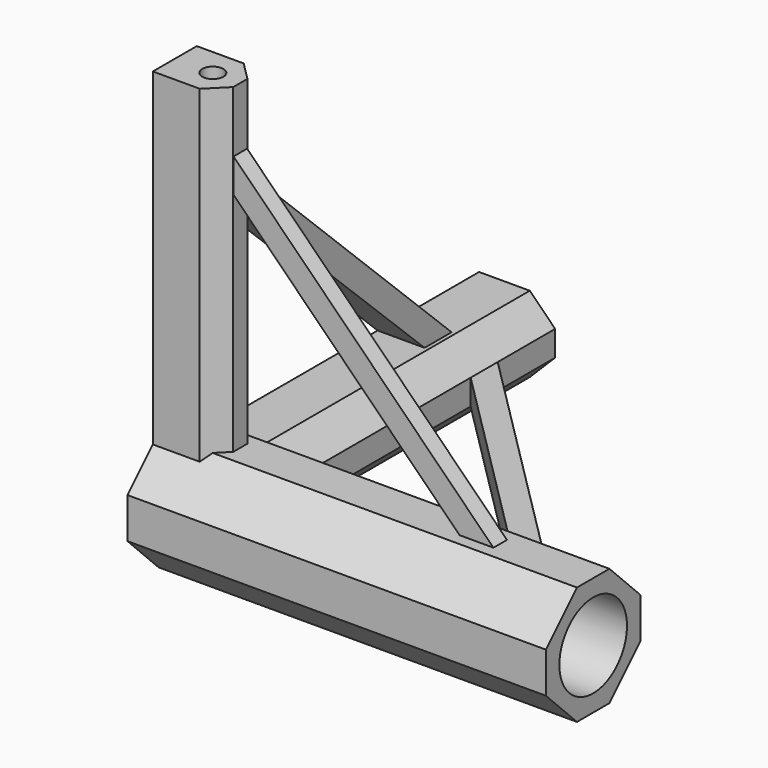
from build123d import *

# Parameters (mm, degrees)
F1_W          = 17.78
F1_H          = 17.78
F2_DEPTH      = 57.15
F4_SIZE       = 5.842
F6_W          = 8.255
F6_H          = 8.255
F7_DEPTH      = 57.15
F8_DEPTH      = 8.89
F10_T4_DEPTH  = 63.7100645368
F10_T9_DEPTH  = 63.7100645368
F10_T14_DEPTH = 15.4500645368
F10_T19_DEPTH = 63.7100645368
F10_T24_DEPTH = 63.7100645368
F10_T29_DEPTH = 15.4500645368
F12_W         = 11.43
F12_H         = 11.43
F13_DEPTH     = 57.15
F15_SIZE      = 3.81
F17_DEPTH     = 1.27
F19_DEPTH     = 1.905
F20_DEPTH     = 5.715
F21_T1_DEPTH  = 35.7625440314
F21_T6_DEPTH  = 35.7625440314
F21_T12_DEPTH = 35.7625440314
F21_T17_DEPTH = 35.7625440314
F21_T22_DEPTH = 35.7625440314
F22_DEPTH     = 1.5875
F25_DEPTH     = 7.0485


# Not quite as in the source:
# - a fillet or chamfer that OpenCascade refuses, or shapes differently, is made with other operations: its cross-section is extruded or revolved along the edge and cut away or added
# - an extrude ends at something that could not be found from the text; its depth is read off the source's solid


with BuildPart() as f2:
    # F1 (on Right) → F2 (new body)
    with BuildSketch(Plane.YZ):
        Rectangle(F1_W, F1_H)
    extrude(amount=F2_DEPTH)

    # F0 (on Front) → F3 (revolve, cut)
    with BuildSketch(Plane.XZ):
        Polygon((11.43, 3.175), (11.43, 0), (62.23, 0), (62.23, 6.35), (14.605, 6.35), align=None)
    revolve(axis=Axis((36.83, 0, 0), (1, 0, 0)), mode=Mode.SUBTRACT)

    # F4
    f4_edges = [f2.edges().sort_by_distance(p)[0] for p in [
        (28.575, -8.89, -8.89),
        (28.575, 8.89, 8.89),
        (28.575, -8.89, 8.89),
        (28.575, 8.89, -8.89),
    ]]
    chamfer(f4_edges, length=F4_SIZE)

    # F6 (on Top) → F7 (join)
    with BuildSketch(Plane.XY):
        Rectangle(F6_W, F6_H)
    extrude(amount=F7_DEPTH)

    # F8 (add, through all): a face of the model
    f8_faces = [f2.faces().sort_by_distance(p)[0] for p in [
        (-2.06375, 0, 0),
    ]]
    extrude(f8_faces, amount=F8_DEPTH)

    # F5 (on Right) → F9 (revolve, cut)
    with BuildSketch(Plane.YZ):
        Polygon((0, 66.04), (0, 11.43), (0.79375, 11.43), (1.5875, 12.22375), (1.5875, 66.04), align=None)
    revolve(axis=Axis((0, 0, 38.735), (0, 0, -1)), mode=Mode.SUBTRACT)

    # F10: chamfer of 2.794 on 4 edges, made by hand


with BuildPart() as f10_tool2:
    # F10_s3 → F10_t4 (new body)
    with BuildSketch(Plane.XY.offset(0.6252177316)):
        Polygon((4.1275, 1.3335), (1.3335, 4.1275), (4.1275, 4.1275), align=None)
    extrude(amount=F10_T4_DEPTH)

    split(bisect_by=Plane(origin=(0, 5.969, 5.969), x_dir=(1, 0, 0), z_dir=(0, 0.7071067812, 0.7071067812)), keep=Keep.TOP)


with BuildPart() as f2_1:
    add(f2.part)

    # F10_t1: cut F10_tool2
    add(f10_tool2.part, mode=Mode.SUBTRACT)


with BuildPart() as f10_tool7:
    # F10_s8 → F10_t9 (new body)
    with BuildSketch(Plane.XY.offset(0.6252177316)):
        Polygon((4.1275, 1.3335), (1.3335, 4.1275), (4.1275, 4.1275), align=None)
    extrude(amount=F10_T9_DEPTH)

    split(bisect_by=Plane.XY.offset(8.89), keep=Keep.TOP)


with BuildPart() as f2_2:
    add(f2_1.part)

    # F10_t6: cut F10_tool7
    add(f10_tool7.part, mode=Mode.SUBTRACT)


with BuildPart() as f10_tool12:
    # F10_s13 → F10_t14 (new body)
    with BuildSketch(Plane.XY.offset(-0.6252177316)):
        Polygon((-2.794, 4.1275), (0, 1.3335), (0, 4.1275), align=None)
    extrude(amount=-F10_T14_DEPTH)

    split(bisect_by=Plane(origin=(0, 5.969, -5.969), x_dir=(1, 0, 0), z_dir=(0, 0.7071067812, -0.7071067812)), keep=Keep.TOP)


with BuildPart() as f2_3:
    add(f2_2.part)

    # F10_t11: cut F10_tool12
    add(f10_tool12.part, mode=Mode.SUBTRACT)


with BuildPart() as f10_tool17:
    # F10_s18 → F10_t19 (new body)
    with BuildSketch(Plane.XY.offset(0.6252177316)):
        Polygon((1.3335, -4.1275), (4.1275, -1.3335), (4.1275, -4.1275), align=None)
    extrude(amount=F10_T19_DEPTH)

    split(bisect_by=Plane.XY.offset(8.89), keep=Keep.TOP)


with BuildPart() as f2_4:
    add(f2_3.part)

    # F10_t16: cut F10_tool17
    add(f10_tool17.part, mode=Mode.SUBTRACT)


with BuildPart() as f10_tool22:
    # F10_s23 → F10_t24 (new body)
    with BuildSketch(Plane.XY.offset(0.6252177316)):
        Polygon((1.3335, -4.1275), (4.1275, -1.3335), (4.1275, -4.1275), align=None)
    extrude(amount=F10_T24_DEPTH)

    split(bisect_by=Plane(origin=(0, -5.969, 5.969), x_dir=(1, 0, 0), z_dir=(0, -0.7071067812, 0.7071067812)), keep=Keep.TOP)


with BuildPart() as f2_5:
    add(f2_4.part)

    # F10_t21: cut F10_tool22
    add(f10_tool22.part, mode=Mode.SUBTRACT)


with BuildPart() as f10_tool27:
    # F10_s28 → F10_t29 (new body)
    with BuildSketch(Plane.XY.offset(-0.6252177316)):
        Polygon((-2.794, -4.1275), (0, -1.3335), (0, -4.1275), align=None)
    extrude(amount=-F10_T29_DEPTH)

    split(bisect_by=Plane(origin=(0, -5.969, -5.969), x_dir=(1, 0, 0), z_dir=(0, -0.7071067812, -0.7071067812)), keep=Keep.TOP)


with BuildPart() as f2_6:
    add(f2_5.part)

    # F10_t26: cut F10_tool27
    add(f10_tool27.part, mode=Mode.SUBTRACT)

    # F12 (on Front) → F13 (join)
    with BuildSketch(Plane.XZ):
        Rectangle(F12_W, F12_H)
    extrude(amount=-F13_DEPTH)

    # F11 (on Top) → F14 (revolve, cut)
    with BuildSketch(Plane.XY):
        Polygon((0, 66.04), (-3.175, 66.04), (-3.175, 13.0175), (-1.5875, 11.43), (0, 11.43), align=None)
    revolve(axis=Axis((0, 24.5966146997, 0), (0, 1, 0)), mode=Mode.SUBTRACT)

    # F15
    f15_edges = [f2_6.edges().sort_by_distance(p)[0] for p in [
        (5.715, 31.6865, 5.715),
        (5.715, 31.6865, -5.715),
        (-5.715, 28.575, -5.715),
    ]]
    chamfer(f15_edges, length=F15_SIZE)

    # F16 (on Front) → F17 (join, symmetric)
    with BuildSketch(Plane.XZ):
        Polygon((43.18, 8.89), (4.1275, 47.9425), (4.1275, 42.8625), (38.1, 8.89), align=None)
    extrude(amount=F17_DEPTH, both=True)

    # F18 (on Top) → F19 (join, symmetric)
    with BuildSketch(Plane.XY):
        Polygon((43.18, 8.89), (5.715, 46.355), (5.715, 41.275), (38.1, 8.89), align=None)
    extrude(amount=F19_DEPTH, both=True)

    # F1 (on Right) → F20 (join, through all)
    with BuildSketch(Plane.YZ):
        Rectangle(F1_W, F1_H)
    extrude(amount=-F20_DEPTH)

    # F21: chamfer of 5.842 on 4 edges, made by hand

    # F21_s2 → F21_t1 (cut)
    with BuildSketch(Plane.YZ.offset(-20.7387720157)):
        Polygon((-3.048, -8.89), (-8.89, -3.048), (-8.89, -8.89), align=None)
    extrude(amount=F21_T1_DEPTH, mode=Mode.SUBTRACT)


with BuildPart() as f21_tool4:
    # F21_s5 → F21_t6 (new body)
    with BuildSketch(Plane.YZ.offset(15.0237720157)):
        Polygon((3.048, 8.89), (8.89, 3.048), (8.89, 8.89), align=None)
    extrude(amount=-F21_T6_DEPTH)

    split(bisect_by=Plane.XZ.offset(-4.1275), keep=Keep.BOTTOM)

    split(bisect_by=Plane.XY.offset(5.715), keep=Keep.TOP)


with BuildPart() as f2_7:
    add(f2_6.part)

    # F21_t3: cut F21_tool4
    add(f21_tool4.part, mode=Mode.SUBTRACT)


with BuildPart() as f21_tool10:
    # F21_s11 → F21_t12 (new body)
    with BuildSketch(Plane.YZ.offset(15.0237720157)):
        Polygon((-3.048, 8.89), (-8.89, 3.048), (-8.89, 8.89), align=None)
    extrude(amount=-F21_T12_DEPTH)

    split(bisect_by=Plane.XZ.offset(4.1275), keep=Keep.TOP)


with BuildPart() as f2_8:
    add(f2_7.part)

    # F21_t9: cut F21_tool10
    add(f21_tool10.part, mode=Mode.SUBTRACT)


with BuildPart() as f21_tool15:
    # F21_s16 → F21_t17 (new body)
    with BuildSketch(Plane.YZ.offset(15.0237720157)):
        Polygon((3.048, -8.89), (8.89, -3.048), (8.89, -8.89), align=None)
    extrude(amount=-F21_T17_DEPTH)

    split(bisect_by=Plane.XY.offset(-5.715), keep=Keep.BOTTOM)


with BuildPart() as f2_9:
    add(f2_8.part)

    # F21_t14: cut F21_tool15
    add(f21_tool15.part, mode=Mode.SUBTRACT)


with BuildPart() as f21_tool20:
    # F21_s21 → F21_t22 (new body)
    with BuildSketch(Plane.YZ.offset(15.0237720157)):
        Polygon((3.048, -8.89), (8.89, -3.048), (8.89, -8.89), align=None)
    extrude(amount=-F21_T22_DEPTH)

    split(bisect_by=Plane(origin=(-3.81, 0, -3.81), x_dir=(0, 1, 0), z_dir=(-0.7071067812, 0, -0.7071067812)), keep=Keep.TOP)


with BuildPart() as f2_10:
    add(f2_9.part)

    # F21_t19: cut F21_tool20
    add(f21_tool20.part, mode=Mode.SUBTRACT)

    # F22 (add, through all): a face of the model
    f22_faces = [f2_10.faces().sort_by_distance(p)[0] for p in [
        (-4.1275, 0, 33.02),
    ]]
    extrude(f22_faces, amount=F22_DEPTH)

    # F24 (on offset) → F25 (join, through all)
    with BuildSketch(Plane(origin=(-5.715, 0, 0), x_dir=(0, -1, 0), z_dir=(-1, 0, 0))):
        Polygon((-43.18, 5.715), (-38.1, 5.715), (-4.1275, 38.1), (-4.1275, 43.18), align=None)
    extrude(amount=-F25_DEPTH)


solid = f2_10.part
